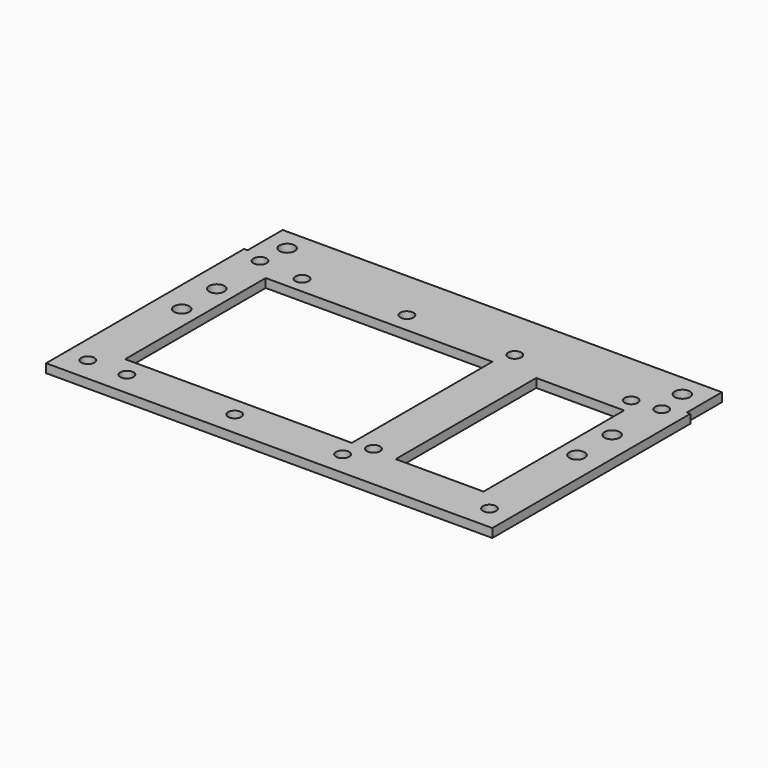
from build123d import *

# Parameters (mm, degrees)
F0_W      = 101.6
F0_H      = 53.34
F1_DEPTH  = 2
F3_D      = 3
F4_W      = 101.6
F4_H      = 3
F4_W_2    = 100
F4_H_2    = 10
F5_DEPTH  = 2
F7_D      = 3.5
F9_D      = 3
F10_W     = 51.6
F10_H     = 40
F10_W_2   = 20
F11_DEPTH = 2.001


with BuildPart() as f1:
    # F0 (on Top) → F1 (new body)
    with BuildSketch(Plane.XY):
        Rectangle(F0_W, F0_H)
    extrude(amount=F1_DEPTH)

    # F3 (through all)
    with Locations(Plane.XY.offset(2)):
        with Locations((-35.56, 24.13), (39.37, 24.13), (45.72, -24.13), (15.24, -19.05), (-36.83, -24.13)):
            Hole(F3_D / 2)

    # F4 (on face) → F5 (join, through all)
    with BuildSketch(Plane.XY.offset(2)):
        with Locations((0, -28.17)):
            Rectangle(F4_W, F4_H)
        with Locations((0, 31.67)):
            Rectangle(F4_W_2, F4_H_2)
    extrude(amount=-F5_DEPTH)

    # F7 (through all)
    with Locations(Plane.XY.offset(2)):
        with Locations((-45, 31.67), (45, 31.67), (-45, 11.67), (-45, 1.67), (45, 11.67), (45, 1.67)):
            Hole(F7_D / 2)

    # F9 (through all)
    with Locations(Plane.XY.offset(2)):
        with Locations((-45.72, -24.13), (-45.72, 24.87), (-12.28, 24.87), (12.28, 24.87), (12.28, -24.13), (-12.28, -24.13), (45.72, 24.87)):
            Hole(F9_D / 2)

    # F10 (on face) → F11 (cut, through all)
    with BuildSketch(Plane(origin=(0, 0, 0), x_dir=(1, 0, 0), z_dir=(0, 0, -1))):
        with Locations((-15, -0.33)):
            Rectangle(F10_W, F10_H)
        with Locations((30.8, -0.33)):
            Rectangle(F10_W_2, F10_H)
    extrude(amount=-F11_DEPTH, mode=Mode.SUBTRACT)


solid = f1.part
